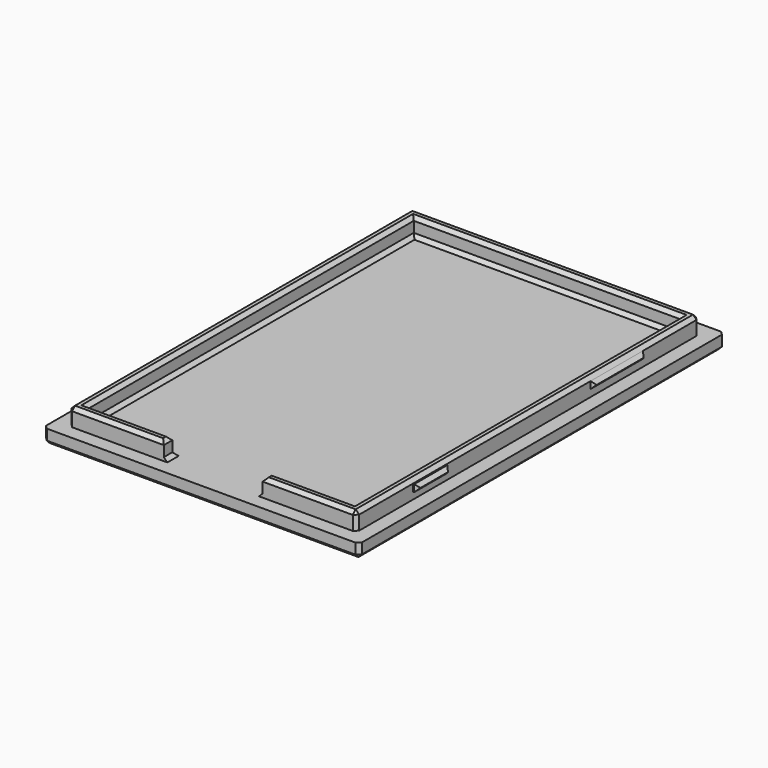
from build123d import *

# Parameters (mm, degrees)
F0_W     = 1.5
F0_H     = 9.3130898729
F0_H_2   = 25.6233112887
F0_H_3   = 5.8635988384
F0_W_2   = 14
F0_H_4   = 2
F0_H_5   = 0.4158456028
F0_W_3   = 0.7
F0_W_4   = 0.5
F0_W_5   = 37.8
F0_H_6   = 8.5
F0_W_6   = 10
F0_H_7   = 1.5
F1_DEPTH = 2
F2_START = 1
F2_DEPTH = 3.5
F3_START = 3
F3_DEPTH = 1
F4_SIZE  = 0.49999


# Not quite as in the source:
# - a fillet or chamfer is up to 0.001 mm smaller than in the source, because OpenCascade refuses the exact size
# - a feature names something its author has since deleted; it is built from what else it names


with BuildPart() as f1:
    # F0 (on Top) → F1 (new body)
    with BuildSketch(Plane.XY):
        Polygon((-20.5, 25.9721875068), (-20.5, 35.9721875068), (20.3, 35.9721875068), (20.3, 25.9721875068), (20.8, 25.9721875068), (20.8, 16.6590976339), (20.3, 16.6590976339), (20.3, -8.9642136547), (21, -8.9642136547), (21, -14.8278124932), (20.3, -14.8278124932), (20.3, -24.8278124932), (17, -24.8278124932), (17, -26.8278124932), (22.3, -26.8278124932), (22.3, -13.9410611472), (22.3, 25.0854361609), (22.3, 37.9721875068), (-22.5, 37.9721875068), (-22.5, 25.0854361609), (-22.5, -13.9410611472), (-22.5, -26.8278124932), (-17, -26.8278124932), (-17, -24.8278124932), (-20.5, -24.8278124932), (-20.5, -14.8278124932), (-21, -14.8278124932), (-21, -8.9642136547), (-20.5, -8.9642136547), (-20.5, 16.6590976339), (-21, 16.6590976339), (-21, 25.9721875068), align=None)
        Polygon((20.3, 35.9721875068), (-20.5, 35.9721875068), (-20.5, 25.9721875068), (-19, 25.9721875068), (-19, 34.4721875068), (18.8, 34.4721875068), (18.8, 25.9721875068), (20.3, 25.9721875068), align=None)
        with Locations((-19.75, 21.3156425704)):
            Rectangle(F0_W, F0_H)
        with Locations((-19.75, 3.8474419896)):
            Rectangle(F0_W, F0_H_2)
        Polygon((18.8, -14.8278124932), (-19, -14.8278124932), (-19, -23.3278124932), (-7, -23.3278124932), (-7, -22.9119668904), (7, -22.9119668904), (7, -23.3278124932), (18.8, -23.3278124932), align=None)
        with Locations((-19.75, -11.8960130739)):
            Rectangle(F0_W, F0_H_3)
        with Locations((0, -25.8278124932)):
            Rectangle(F0_W_2, F0_H_4)
        with Locations((0, -23.1198896918)):
            Rectangle(F0_W_2, F0_H_5)
        Polygon((-19, -14.8278124932), (-20.5, -14.8278124932), (-20.5, -24.8278124932), (-17, -24.8278124932), (-7, -24.8278124932), (-7, -23.3278124932), (-19, -23.3278124932), align=None)
        with Locations((20.65, -11.8960130739)):
            Rectangle(F0_W_3, F0_H_3)
        with Locations((-20.75, -11.8960130739)):
            Rectangle(F0_W_4, F0_H_3)
        with Locations((-20.75, 21.3156425704)):
            Rectangle(F0_W_4, F0_H)
        with Locations((20.55, 21.3156425704)):
            Rectangle(F0_W_4, F0_H)
        with Locations((-0.1, 30.2221875068)):
            Rectangle(F0_W_5, F0_H_6)
        with Locations((-0.1, 21.3156425704)):
            Rectangle(F0_W_5, F0_H)
        with Locations((-0.1, 3.8474419896)):
            Rectangle(F0_W_5, F0_H_2)
        with Locations((-0.1, -11.8960130739)):
            Rectangle(F0_W_5, F0_H_3)
        with Locations((-12, -25.8278124932)):
            Rectangle(F0_W_6, F0_H_4)
        with Locations((0, -24.0778124932)):
            Rectangle(F0_W_2, F0_H_7)
        Polygon((20.3, -24.8278124932), (20.3, -14.8278124932), (18.8, -14.8278124932), (18.8, -23.3278124932), (7, -23.3278124932), (7, -24.8278124932), (17, -24.8278124932), align=None)
        with Locations((12, -25.8278124932)):
            Rectangle(F0_W_6, F0_H_4)
        with Locations((19.55, -11.8960130739)):
            Rectangle(F0_W, F0_H_3)
        with Locations((19.55, 3.8474419896)):
            Rectangle(F0_W, F0_H_2)
        with Locations((19.55, 21.3156425704)):
            Rectangle(F0_W, F0_H)
    extrude(amount=F1_DEPTH)

    # F0 (on Top) → F2 (join)
    with BuildSketch(Plane.XY.offset(F2_START)):
        Polygon((20.3, 35.9721875068), (-20.5, 35.9721875068), (-20.5, 25.9721875068), (-19, 25.9721875068), (-19, 34.4721875068), (18.8, 34.4721875068), (18.8, 25.9721875068), (20.3, 25.9721875068), align=None)
        with Locations((-19.75, 21.3156425704)):
            Rectangle(F0_W, F0_H)
        with Locations((-19.75, 3.8474419896)):
            Rectangle(F0_W, F0_H_2)
        with Locations((19.55, 21.3156425704)):
            Rectangle(F0_W, F0_H)
        with Locations((19.55, 3.8474419896)):
            Rectangle(F0_W, F0_H_2)
        Polygon((20.3, -24.8278124932), (20.3, -14.8278124932), (18.8, -14.8278124932), (18.8, -23.3278124932), (7, -23.3278124932), (7, -24.8278124932), (17, -24.8278124932), align=None)
        with Locations((19.55, -11.8960130739)):
            Rectangle(F0_W, F0_H_3)
        Polygon((-19, -14.8278124932), (-20.5, -14.8278124932), (-20.5, -24.8278124932), (-17, -24.8278124932), (-7, -24.8278124932), (-7, -23.3278124932), (-19, -23.3278124932), align=None)
        with Locations((-19.75, -11.8960130739)):
            Rectangle(F0_W, F0_H_3)
    extrude(amount=F2_DEPTH)

    # F0 (on Top) → F3 (join)
    with BuildSketch(Plane.XY.offset(F3_START)):
        with Locations((20.55, 21.3156425704)):
            Rectangle(F0_W_4, F0_H)
        with Locations((-20.75, 21.3156425704)):
            Rectangle(F0_W_4, F0_H)
        with Locations((-20.75, -11.8960130739)):
            Rectangle(F0_W_4, F0_H_3)
        with Locations((20.65, -11.8960130739)):
            Rectangle(F0_W_3, F0_H_3)
    extrude(amount=F3_DEPTH)

    # F4 (size 0.5 in the source; OpenCascade refuses exactly that, so slightly less here)
    f4_edges = [f1.edges().sort_by_distance(p)[0] for p in [
        (-21, 25.972188, 3.5),
        (-21, 16.659098, 3.5),
        (-21, 21.315643, 3),
        (-21, 21.315643, 4),
        (-21, -8.964214, 3.5),
        (-21, -14.827812, 3.5),
        (-21, -11.896013, 3),
        (-21, -11.896013, 4),
        (20.8, 16.659098, 3.5),
        (20.8, 25.972188, 3.5),
        (20.8, 21.315643, 3),
        (20.8, 21.315643, 4),
        (21, -14.827812, 3.5),
        (21, -8.964214, 3.5),
        (21, -11.896013, 3),
        (21, -11.896013, 4),
        (20.3, -24.827812, 3.25),
        (20.3, 35.972188, 3.25),
        (-0.1, 35.972188, 4.5),
        (-20.5, 5.572188, 4.5),
        (-13.75, -24.827812, 4.5),
        (-7, -24.077812, 4.5),
        (-13, -23.327812, 4.5),
        (-19, 5.572188, 4.5),
        (-0.1, 34.472188, 4.5),
        (18.8, 5.572188, 4.5),
        (12.9, -23.327812, 4.5),
        (7, -24.077812, 4.5),
        (13.65, -24.827812, 4.5),
        (20.3, 5.572188, 4.5),
        (-20.5, 35.972188, 3.25),
        (-22.5, 37.972188, 1),
        (-20.5, -24.827812, 3.25),
        (-22.5, -26.827812, 1),
        (22.3, -26.827812, 1),
        (22.3, 5.572188, 0),
        (-0.1, 37.972188, 0),
        (-22.5, 5.572188, 0),
        (-0.1, -26.827812, 0),
        (12.9, -23.327812, 2),
        (18.8, 5.572188, 2),
        (-13, -23.327812, 2),
        (-19, 5.572188, 2),
        (-0.1, 34.472188, 2),
        (7, -24.077812, 2),
        (-7, -24.077812, 2),
        (22.3, 37.972188, 1),
    ]]
    chamfer(f4_edges, length=F4_SIZE)


solid = f1.part
